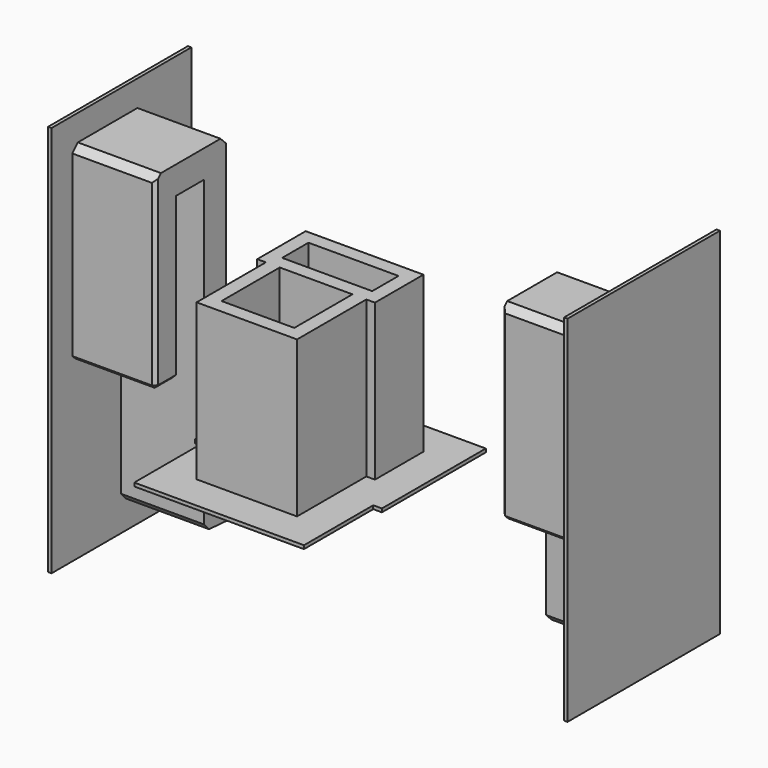
from build123d import *

# Parameters (mm, degrees)
F1_DEPTH    = 16
F0_W        = 8.4
F0_H        = 8.4
F0_R        = 1.9
F2_DEPTH    = 2.4
F4_W        = 3.6
F4_H        = 3.2
F5_DEPTH    = 5
F6_T1_DEPTH = 14.1146927807
F6_T3_DEPTH = 13.8486241795
F8_W        = 3
F8_H        = 3.2
F8_W_2      = 1.4
F9_DEPTH    = 5
F10_SIZE    = 0.8
F12_SIZE    = 0.4
F12_2_SIZE  = 0.4
F13_SIZE    = 0.4
F14_W       = 4
F14_H       = 0.4
F16_W       = 20.190256201
F16_H       = 45.2759127293
F17_DEPTH   = 0.4
F18_W       = 22.0095793974
F18_H       = 41
F19_DEPTH   = 0.4


# Not quite as in the source:
# - a fillet or chamfer that OpenCascade refuses, or shapes differently, is made with other operations: its cross-section is extruded or revolved along the edge and cut away or added
# - a feature names something its author has since deleted; it is built from what else it names


with BuildPart() as f1:
    # F0 (on Top) → F1 (new body)
    with BuildSketch(Plane.XY):
        Polygon((-5.8, 4.2), (-4.2, 4.2), (4.2, 4.2), (5.8, 4.2), (5.8, 5.8), (5.2, 5.8), (-5.2, 5.8), (-5.8, 5.8), align=None)
        Polygon((-4.2, -4.2), (-4.2, 4.2), (-5.8, 4.2), (-5.8, -5.8), (5.8, -5.8), (5.8, 4.2), (4.2, 4.2), (4.2, -4.2), align=None)
        Polygon((-6.8, 4.2), (-5.8, 4.2), (-5.8, 5.8), (-5.2, 5.8), (-5.2, 9.6), (5.2, 9.6), (5.2, 5.8), (5.8, 5.8), (5.8, 4.2), (6.8, 4.2), (6.8, 11.2), (-6.8, 11.2), align=None)
    extrude(amount=F1_DEPTH)

    # F0 (on Top) → F2 (join)
    with BuildSketch(Plane.XY):
        Polygon((-5.8, 4.2), (-4.2, 4.2), (4.2, 4.2), (5.8, 4.2), (5.8, 5.8), (5.2, 5.8), (-5.2, 5.8), (-5.8, 5.8), align=None)
        Rectangle(F0_W, F0_H)
        Circle(F0_R, mode=Mode.SUBTRACT)
        Polygon((-6.8, 4.2), (-5.8, 4.2), (-5.8, 5.8), (-5.2, 5.8), (-5.2, 9.6), (5.2, 9.6), (5.2, 5.8), (5.8, 5.8), (5.8, 4.2), (6.8, 4.2), (6.8, 11.2), (-6.8, 11.2), align=None)
        Polygon((-4.2, -4.2), (-4.2, 4.2), (-5.8, 4.2), (-5.8, -5.8), (5.8, -5.8), (5.8, 4.2), (4.2, 4.2), (4.2, -4.2), align=None)
    extrude(amount=-F2_DEPTH)

    # F13
    f13_edges = [f1.edges().sort_by_distance(p)[0] for p in [
        (-1.9, 0, -2.4),
    ]]
    chamfer(f13_edges, length=F13_SIZE)

    # F15: sweep along a path in F15_path
    with BuildLine(Plane(origin=(-5.8, 4.2, -2.4), x_dir=(0, 1, 0), z_dir=(0, 0, 1))) as f15_path:
        Line((0, 0), (-10, 0))
        Line((-10, 0), (-10, -11.6))
        Line((-10, -11.6), (0, -11.6))
        Line((0, -11.6), (0, -12.6))
        Line((0, -12.6), (7, -12.6))
        Line((7, -12.6), (7, 1))
        Line((7, 1), (0, 1))
        Line((0, 1), (0, 0))
    # F14 (on Front) → F15 (sweep)
    with BuildSketch(Plane.XZ):
        with Locations((-7.8, -2.2)):
            Rectangle(F14_W, F14_H)
    sweep(path=f15_path.line, transition=Transition.RIGHT)


with BuildPart() as f5:
    # F4 (on offset) → F5 (new body, symmetric)
    with BuildSketch(Plane.YZ.offset(-25)):
        Polygon((6, 19.4), (6, -2.4), (9.4, -2.4), (9.4, 16.2), (9.4, 19.4), align=None)
        Polygon((13, 19.4), (13, 16.2), (13, -16.6), (14.5960929631, -16.6), (14.8271182356, -13.2961846812), (16.2, -13.3921859261), (16.2, -12.9097403669), (16.2, 19.4), align=None)
        with Locations((11.2, 17.8)):
            Rectangle(F4_W, F4_H)
        Polygon((14.8271182356, -13.2961846812), (14.5960929631, -16.6), (16.2, -16.6), (16.2, -13.3921859261), align=None)
        Polygon((16.2, -16.6), (14.5960929631, -16.6), (14.3806768036, -19.6805946028), (19.9670354851, -20.0712308558), (20.413476917, -13.6868209341), (18.8173744366, -13.5752105762), (18.5941537206, -16.767415537), align=None)
        Polygon((14.5960929631, -16.6), (13, -16.6), (14.3806768036, -19.6805946028), align=None)
        Polygon((16.2, -13.3921859261), (16.2, -16.6), (16.423220716, -13.4077950392), align=None)
        Polygon((16.423220716, -13.4077950392), (16.2, -12.9097403669), (16.2, -13.3921859261), align=None)
        Polygon((14.3806768036, -19.6805946028), (13, -16.6), (13, -19.5840482756), align=None)
    extrude(amount=F5_DEPTH, both=True)

    # F6: chamfer of 0.8 on 5 edges, made by hand

    # F6_s2 → F6_t1 (cut)
    with BuildSketch(Plane.YZ.offset(-32.0573463904)):
        Polygon((20.0228406641, -19.2731796156), (19.1689842449, -20.0154256768), (19.9670354851, -20.0712308558), align=None)
        Polygon((19.6154256768, -13.6310157551), (20.357671738, -14.4848721744), (20.413476917, -13.6868209341), align=None)
        Polygon((15.4, 19.4), (16.2, 18.6), (16.2, 19.4), align=None)
        Polygon((6, 18.6), (6.8, 19.4), (6, 19.4), align=None)
    extrude(amount=F6_T1_DEPTH, mode=Mode.SUBTRACT)

    # F6_s4 → F6_t3 (cut)
    with BuildSketch(Plane.YZ.offset(-31.9243120897)):
        Polygon((13.744194821, -19.6360874469), (13, -18.8380362067), (13, -19.5840482756), align=None)
    extrude(amount=F6_T3_DEPTH, mode=Mode.SUBTRACT)

    # F12
    f12_edges = [f5.edges().sort_by_distance(p)[0] for p in [
        (-25, 6, -2.4),
        (-20, 7.7, -2.4),
        (-25, 9.4, -2.4),
        (-20, 9.4, 6.9),
        (-20, 6, 8.1),
    ]]
    chamfer(f12_edges, length=F12_SIZE)

    # F16 (on face) → F17 (join)
    with BuildSketch(Plane(origin=(-30, 0, 0), x_dir=(0, -1, 0), z_dir=(-1, 0, 0))):
        with Locations((-13.0951281005, -0.2379563647)):
            Rectangle(F16_W, F16_H)
    extrude(amount=-F17_DEPTH)


with BuildPart() as f9:
    # F8 (on offset) → F9 (new body, symmetric)
    with BuildSketch(Plane.YZ.offset(25)):
        Polygon((9.4, 16.2), (9.4, 19.4), (6, 19.4), (6, -2.4), (9.4, -2.4), align=None)
        with Locations((10.9, 17.8)):
            Rectangle(F8_W, F8_H)
        Polygon((14.8, 19.4), (12.4, 19.4), (12.4, 16.2), (12.4, -15.6), (14.8, -15.6), (14.8, -12.4), align=None)
        with Locations((15.5, -14)):
            Rectangle(F8_W_2, F8_H)
        Polygon((16.2, 5.4), (16.2, -12.4), (16.2, -15.6), (18.6, -15.6), (18.6, 5.2321756513), align=None)
        Polygon((18.6, 5.4), (16.2, 5.4), (18.6, 5.2321756513), align=None)
        Polygon((16.646441432, 11.7844099217), (16.2, 5.4), (18.6, 5.4), (18.6, 5.2321756513), (21.7863586815, 5.009363747), (22.2328001134, 11.3937736687), (20.636697633, 11.5053840267), (20.413476917, 8.3131790659), (18.0193231964, 8.4805946028), (18.2425439124, 11.6727995637), align=None)
    extrude(amount=F9_DEPTH, both=True)

    # F10
    f10_edges = [f9.edges().sort_by_distance(p)[0] for p in [
        (25, 22.2328, 11.393774),
        (25, 21.786359, 5.009364),
        (25, 16.646441, 11.78441),
        (25, 6, 19.4),
        (25, 14.8, 19.4),
        (25, 18.6, -15.6),
        (25, 12.4, -15.6),
    ]]
    chamfer(f10_edges, length=F10_SIZE)

    # F12#2
    f12_2_edges = [f9.edges().sort_by_distance(p)[0] for p in [
        (20, 6, 8.1),
        (25, 6, -2.4),
        (20, 7.7, -2.4),
        (25, 9.4, -2.4),
        (20, 9.4, 6.9),
    ]]
    chamfer(f12_2_edges, length=F12_2_SIZE)

    # F18 (on face) → F19 (join)
    with BuildSketch(Plane.YZ.offset(30)):
        with Locations((14.0047896987, 1.9)):
            Rectangle(F18_W, F18_H)
    extrude(amount=-F19_DEPTH)


solid = Compound([f1.part, f5.part, f9.part])
